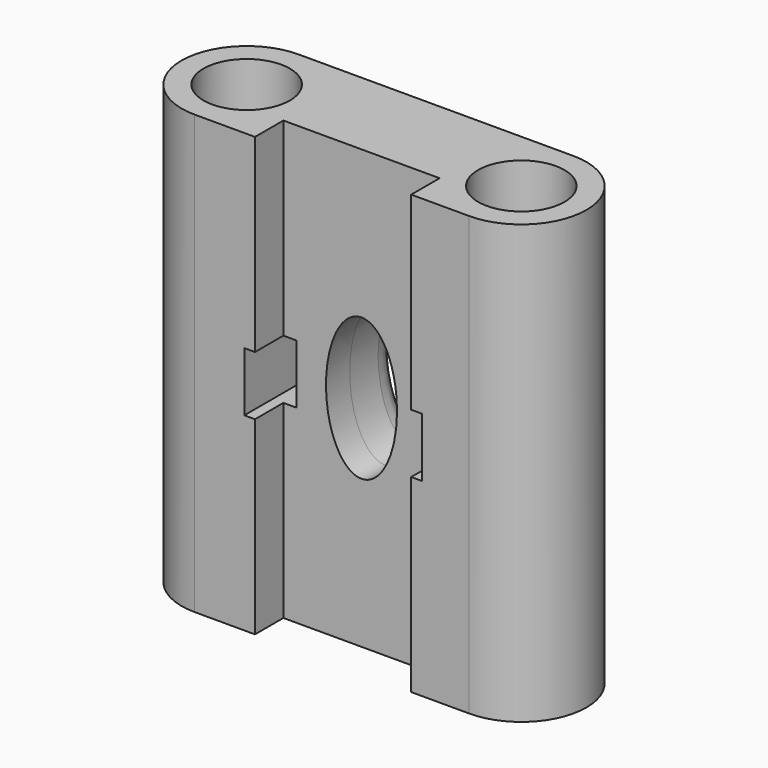
from build123d import *

# Parameters (mm, degrees)
F0_R          = 3.65
F1_DEPTH      = 37
F2_W          = 2
F2_H          = 5
F3_DEPTH      = 20
F3_DEPTH_BACK = 20
F4_R          = 2.5


with BuildPart() as f1:
    # F0 (on Top) → F1 (new body)
    with BuildSketch(Plane.XY):
        with BuildLine():
            Line((11.5, 5.5), (-11.7, 5.5))
            ThreePointArc((-11.7, 5.5), (-17.2, 0), (-11.7, -5.5))
            Line((-11.7, -5.5), (-6.6, -5.5))
            Line((-6.6, -5.5), (-6.6, -2.5))
            Line((-6.6, -2.5), (6.6, -2.5))
            Line((6.6, -2.5), (6.6, -5.5))
            Line((6.6, -5.5), (11.5, -5.5))
            ThreePointArc((11.5, -5.5), (17, 0), (11.5, 5.5))
        make_face()
        with Locations((-11.7, 0)):
            Circle(F0_R, mode=Mode.SUBTRACT)
        with Locations((11.5, 0)):
            Circle(F0_R, mode=Mode.SUBTRACT)
    extrude(amount=F1_DEPTH)

    # F2 (on Front) → F3 (cut, two sides)
    with BuildSketch(Plane.XZ) as f3_sk:
        with Locations((-6.5, 18.5)):
            Rectangle(F2_W, F2_H)
        with Locations((6.5, 18.5)):
            Rectangle(F2_W, F2_H)
        with BuildLine():
            add(Edge.make_bspline(
                [(0, 12.5), (5.1961524227, 12.5), (2.5980762114, 21.5), (0, 30.5), (-2.5980762114, 21.5), (-5.1961524227, 12.5), (0, 12.5)],
                knots=[0, 0, 0, 2.0943951024, 2.0943951024, 4.1887902048, 4.1887902048, 6.2831853072, 6.2831853072, 6.2831853072], degree=2, weights=[1, 0.5, 1, 0.5, 1, 0.5, 1]))
        make_face()
    extrude(amount=F3_DEPTH, mode=Mode.SUBTRACT)
    extrude(f3_sk.sketch, amount=-F3_DEPTH_BACK, mode=Mode.SUBTRACT)

    # F4
    f4_edges = [f1.edges().sort_by_distance(p)[0] for p in [
        (0, 5.5, 24.5),
    ]]
    fillet(f4_edges, radius=F4_R)


solid = f1.part
